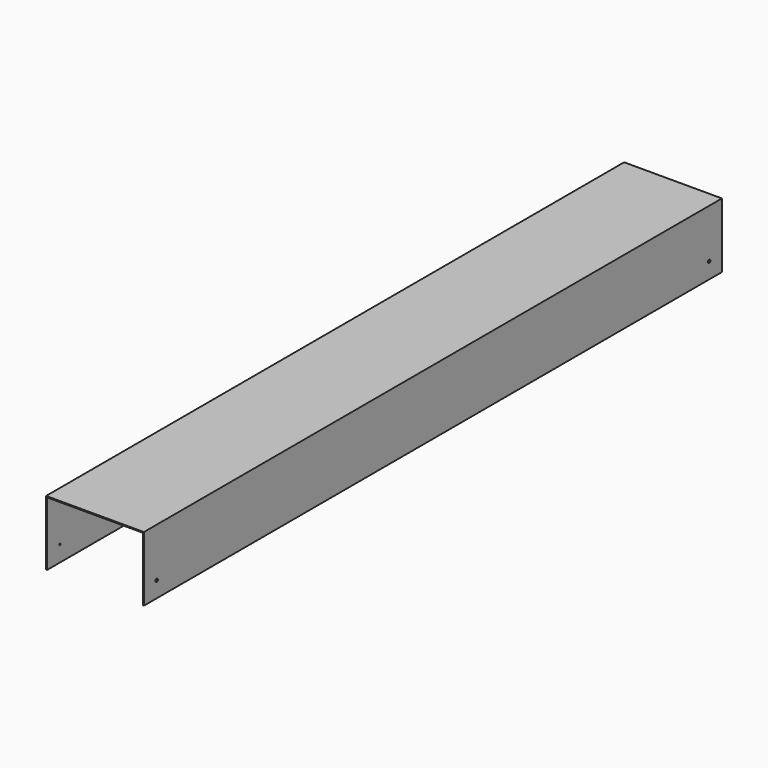
from build123d import *

# Parameters (mm, degrees)
F1_DEPTH         = 1149.35
F3_D             = 4.7625
F3_DEPTH         = 25.4
F3_CSINK_D       = 9.525
F3_CSINK_ANGLE   = 90
F3_TIP           = 1.4307993491
F3_COPIES2_COUNT = 2


# Not quite as in the source:
# - a pattern or mirror of a feature is missing from the dataset's text; its kind, count and spacing are read off the source's solid


with BuildPart() as f1:
    # F0 (on Front) → F1 (new body, symmetric)
    with BuildSketch(Plane.XZ):
        Polygon((155.575, -103.1875), (155.575, 103.1875), (-155.575, 103.1875), (-155.575, -103.1875), (-152.4, -103.1875), (-152.4, 100.0125), (152.4, 100.0125), (152.4, -103.1875), align=None)
    extrude(amount=F1_DEPTH, both=True)

    # F3
    with Locations(Plane.YZ.offset(155.575)):
        with Locations((-1098.55, -52.3875)):
            f3 = CounterSinkHole(F3_D / 2, F3_CSINK_D / 2, depth=F3_DEPTH, counter_sink_angle=F3_CSINK_ANGLE)
            with Locations((0, 0, -(F3_DEPTH + F3_TIP / 2))):  # 118° drill point
                Cone(0, F3_D / 2, F3_TIP, mode=Mode.SUBTRACT)

    # F3_copies: F3 across plane
    add(f3.mirror(Plane(origin=(0, 0, 0), x_dir=(0, 0, -1), z_dir=(-1, 0, 0))), mode=Mode.SUBTRACT)

    # F3_copies1: F3 across plane
    add(f3.mirror(Plane.ZX), mode=Mode.SUBTRACT)

    # F3_copies2: F3 ×2 about axis
    f3_copies2_axis = Axis((0, 0, 0), (0, 0, 1))
    for i in range(1, F3_COPIES2_COUNT):
        add(f3.rotate(f3_copies2_axis, i * 360 / F3_COPIES2_COUNT), mode=Mode.SUBTRACT)


solid = f1.part
